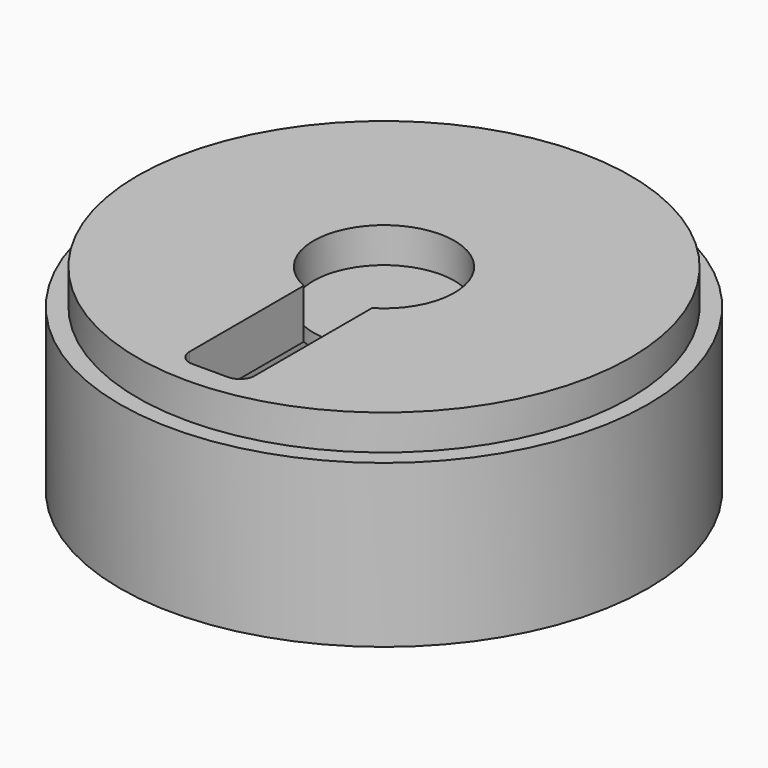
from build123d import *

# Parameters (mm, degrees)
F0_R      = 37.5
F1_DEPTH  = 28
F2_W      = 33
F2_H      = 63
F3_DEPTH  = 21
F4_R      = 10
F5_DEPTH  = 5
F7_DEPTH  = 25
F9_DEPTH  = 15
F10_R     = 37.5
F10_R_2   = 35
F11_DEPTH = 5


with BuildPart() as f1:
    # F0 (on Top) → F1 (new body)
    with BuildSketch(Plane.XY):
        Circle(F0_R)
    extrude(amount=F1_DEPTH)

    # F2 (on face) → F3 (cut)
    with BuildSketch(Plane(origin=(0, 0, 0), x_dir=(1, 0, 0), z_dir=(0, 0, -1))):
        Rectangle(F2_W, F2_H)
    extrude(amount=-F3_DEPTH, mode=Mode.SUBTRACT)

    # F4 (on face) → F5 (cut)
    with BuildSketch(Plane.XY.offset(28)):
        Circle(F4_R)
    extrude(amount=-F5_DEPTH, mode=Mode.SUBTRACT)

    # F6 (on face) → F7 (cut)
    with BuildSketch(Plane(origin=(0, 0, 21), x_dir=(1, 0, 0), z_dir=(0, 0, -1))):
        with BuildLine():
            Line((3.0463133007, 31.5), (-1.9864209462, 31.5))
            ThreePointArc((-1.9864209462, 31.5), (-4.0973785389, 29.3890424073), (-1.9864209462, 27.2780848145))
            Line((-1.9864209462, 27.2780848145), (3.0463133007, 27.2780848145))
            ThreePointArc((3.0463133007, 27.2780848145), (5.1572708935, 29.3890424073), (3.0463133007, 31.5))
        make_face()
    extrude(amount=-F7_DEPTH, mode=Mode.SUBTRACT)

    # F8 (on face) → F9 (cut)
    with BuildSketch(Plane.XY.offset(28)):
        with BuildLine():
            Line((-4.0973785389, -9.1220331675), (-4.0973785389, -29.3890424073))
            ThreePointArc((-4.0973785389, -29.3890424073), (-3.4790933748, -27.8963699787), (-1.9864209462, -27.2780848145))
            Line((-1.9864209462, -27.2780848145), (3.0463133007, -27.2780848145))
            ThreePointArc((3.0463133007, -27.2780848145), (4.5389857293, -27.8963699787), (5.1572708935, -29.3890424073))
            Line((5.1572708935, -29.3890424073), (5.1572708935, -8.5675292198))
            ThreePointArc((5.1572708935, -8.5675292198), (0.5980899663, -9.9820983962), (-4.0973785389, -9.1220331675))
        make_face()
    extrude(amount=-F9_DEPTH, mode=Mode.SUBTRACT)

    # F10 (on face) → F11 (cut)
    with BuildSketch(Plane.XY.offset(28)):
        Circle(F10_R)
        Circle(F10_R_2, mode=Mode.SUBTRACT)
    extrude(amount=-F11_DEPTH, mode=Mode.SUBTRACT)


solid = f1.part
